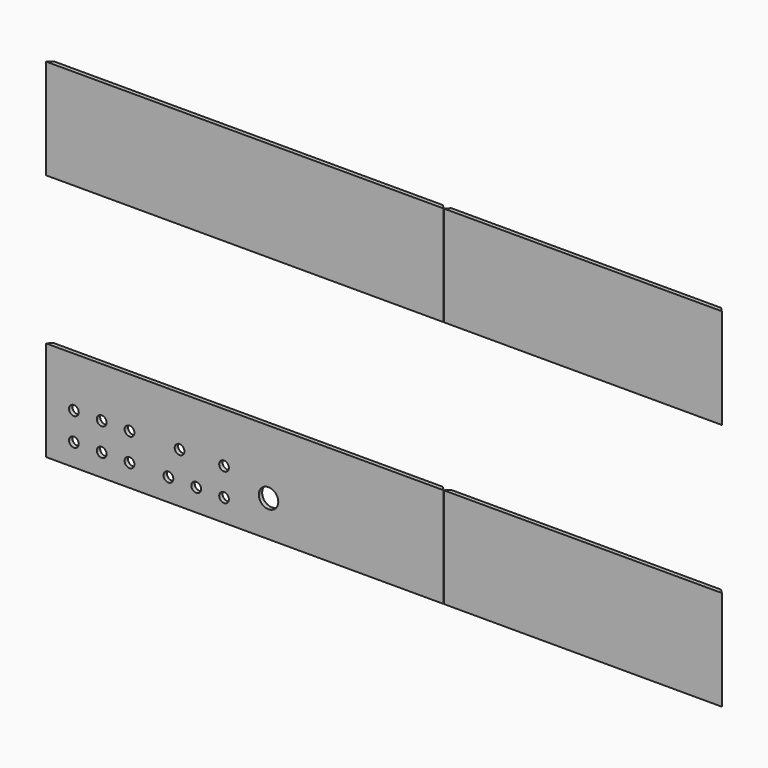
from build123d import *

# Parameters (mm, degrees)
F0_W      = 454.025
F0_H      = 114.3
F0_R      = 5.5626
F0_R_2    = 11.1125
F1_DEPTH  = 4.7752
F0_W_2    = 317.5
F2_SIZE   = 4.77519
F2_2_SIZE = 4.77519
F2_3_SIZE = 4.77519
F2_4_SIZE = 4.77519


# Not quite as in the source:
# - a fillet or chamfer is up to 0.001 mm smaller than in the source, because OpenCascade refuses the exact size
# - a feature names something its author has since deleted; it is built from what else it names


with BuildPart() as f1:
    # F0 (on Front) → F1 (new body)
    with BuildSketch(Plane.XZ):
        with Locations((37.6425363503, 2.1368730813)):
            Rectangle(F0_W, F0_H)
        with Locations((-157.6199636497, -29.6131269187)):
            Circle(F0_R, mode=Mode.SUBTRACT)
        with Locations((-125.8699636497, -29.6131269187)):
            Circle(F0_R, mode=Mode.SUBTRACT)
        with Locations((-94.1199636497, -29.6131269187)):
            Circle(F0_R, mode=Mode.SUBTRACT)
        with Locations((-49.6699636497, -29.6131269187)):
            Circle(F0_R, mode=Mode.SUBTRACT)
        with Locations((-17.9199636497, -29.6131269187)):
            Circle(F0_R, mode=Mode.SUBTRACT)
        with Locations((-157.6199636497, 2.1368730813)):
            Circle(F0_R, mode=Mode.SUBTRACT)
        with Locations((-125.8699636497, 2.1368730813)):
            Circle(F0_R, mode=Mode.SUBTRACT)
        with Locations((-94.1199636497, 2.1368730813)):
            Circle(F0_R, mode=Mode.SUBTRACT)
        with Locations((-36.9699636497, 2.1368730813)):
            Circle(F0_R, mode=Mode.SUBTRACT)
        with Locations((13.8300363503, -29.6131269187)):
            Circle(F0_R, mode=Mode.SUBTRACT)
        with Locations((64.6300363503, -13.7381269187)):
            Circle(F0_R_2, mode=Mode.SUBTRACT)
        with Locations((13.8300363503, 2.1368730813)):
            Circle(F0_R, mode=Mode.SUBTRACT)
    extrude(amount=F1_DEPTH)

    # F2#2 (size 4.7752 in the source; OpenCascade refuses exactly that, so slightly less here)
    f2_2_edges = [f1.edges().sort_by_distance(p)[0] for p in [
        (264.655036, 0, 2.136873),
        (-189.369964, 0, 2.136873),
    ]]
    chamfer(f2_2_edges, length=F2_2_SIZE)


with BuildPart() as f1b:
    # F0 (on Front) → F1, piece 2 (new body)
    with BuildSketch(Plane.XZ):
        with Locations((37.6425363503, 285.3470083714)):
            Rectangle(F0_W, F0_H)
    extrude(amount=F1_DEPTH)

    # F2 (size 4.7752 in the source; OpenCascade refuses exactly that, so slightly less here)
    f2_edges = [f1b.edges().sort_by_distance(p)[0] for p in [
        (264.655036, 0, 285.347008),
        (-189.369964, 0, 285.347008),
    ]]
    chamfer(f2_edges, length=F2_SIZE)


with BuildPart() as f1c:
    # F0 (on Front) → F1, piece 3 (new body)
    with BuildSketch(Plane.XZ):
        with Locations((423.5320413113, 2.1368730813)):
            Rectangle(F0_W_2, F0_H)
    extrude(amount=F1_DEPTH)

    # F2#3 (size 4.7752 in the source; OpenCascade refuses exactly that, so slightly less here)
    f2_3_edges = [f1c.edges().sort_by_distance(p)[0] for p in [
        (582.282041, 0, 2.136873),
        (264.782041, 0, 2.136873),
    ]]
    chamfer(f2_3_edges, length=F2_3_SIZE)


with BuildPart() as f1d:
    # F0 (on Front) → F1, piece 4 (new body)
    with BuildSketch(Plane.XZ):
        with Locations((423.4609160386, 285.3470083714)):
            Rectangle(F0_W_2, F0_H)
    extrude(amount=F1_DEPTH)

    # F2#4 (size 4.7752 in the source; OpenCascade refuses exactly that, so slightly less here)
    f2_4_edges = [f1d.edges().sort_by_distance(p)[0] for p in [
        (264.710916, 0, 285.347008),
        (582.210916, 0, 285.347008),
    ]]
    chamfer(f2_4_edges, length=F2_4_SIZE)


solid = Compound([f1.part, f1b.part, f1c.part, f1d.part])
